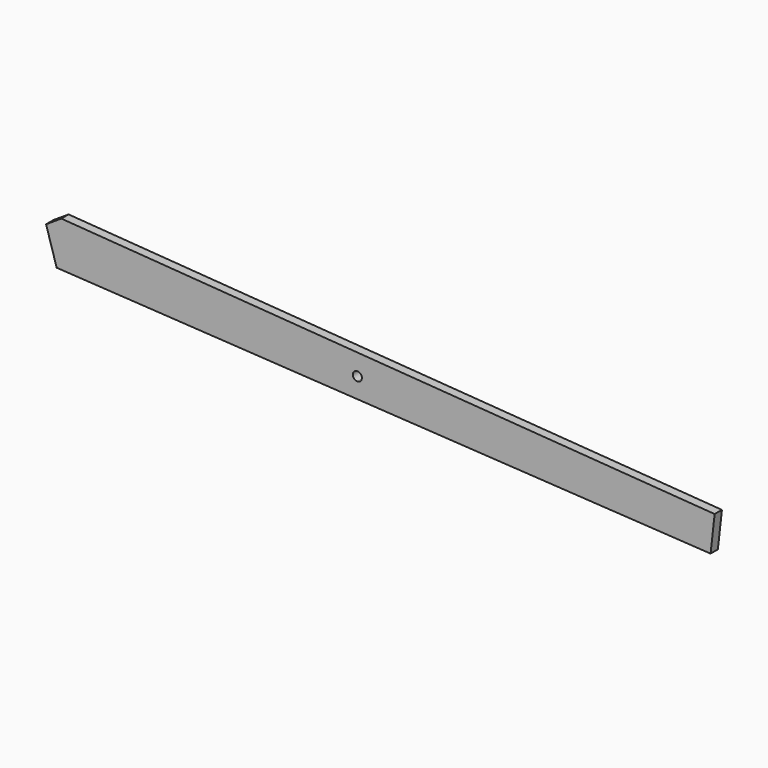
from build123d import *

# Parameters (mm, degrees)
F1_DEPTH = 6.35
F3_D     = 6.35


# Not quite as in the source:
# - a length typed as a fraction of an inch, garbled in the dataset ("3 / 203.2 mm" for 3/8 in), is restored


with BuildPart() as f1:
    # F0 (on Front) → F1 (new body)
    with BuildSketch(Plane.XZ):
        Polygon((-242.4979480523, 80.6390420482), (-253.1238703477, 73.6834848906), (-245.7222477886, 49.3858310226), (210.6660933021, 22.1549273185), (213.4919888436, 47.3972393043), align=None)
    extrude(amount=F1_DEPTH)

    # F3 (through all)
    with Locations(Plane.XZ.offset(6.35)):
        with Locations((-35.8659252524, 50.9419701993)):
            Hole(F3_D / 2)


solid = f1.part
